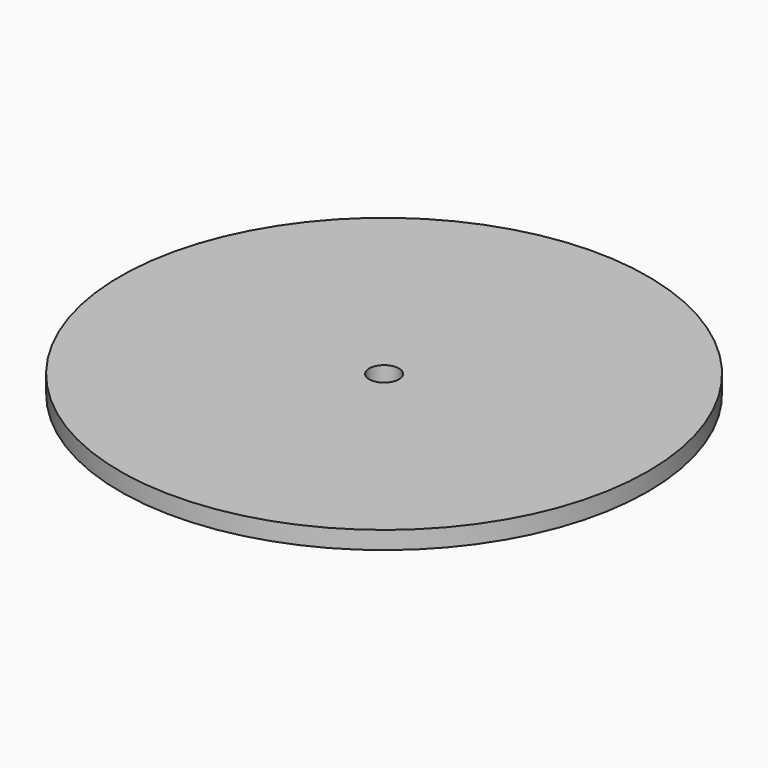
from build123d import *

# Parameters (mm, degrees)
F0_R     = 148.5
F0_R_2   = 8.3312
F1_DEPTH = 10
F2_R     = 146.5
F2_R_2   = 142
F3_DEPTH = 5


# Not quite as in the source:
# - a feature names something its author has since deleted; it is built from what else it names


with BuildPart() as f1:
    # F0 (on Top) → F1 (new body)
    with BuildSketch(Plane.XY):
        Circle(F0_R)
        Circle(F0_R_2, mode=Mode.SUBTRACT)
    extrude(amount=F1_DEPTH)

    # F2 (on face) → F3 (cut)
    with BuildSketch(Plane.XY):
        Circle(F2_R)
        Circle(F2_R_2, mode=Mode.SUBTRACT)
    extrude(amount=F3_DEPTH, mode=Mode.SUBTRACT)


solid = f1.part
